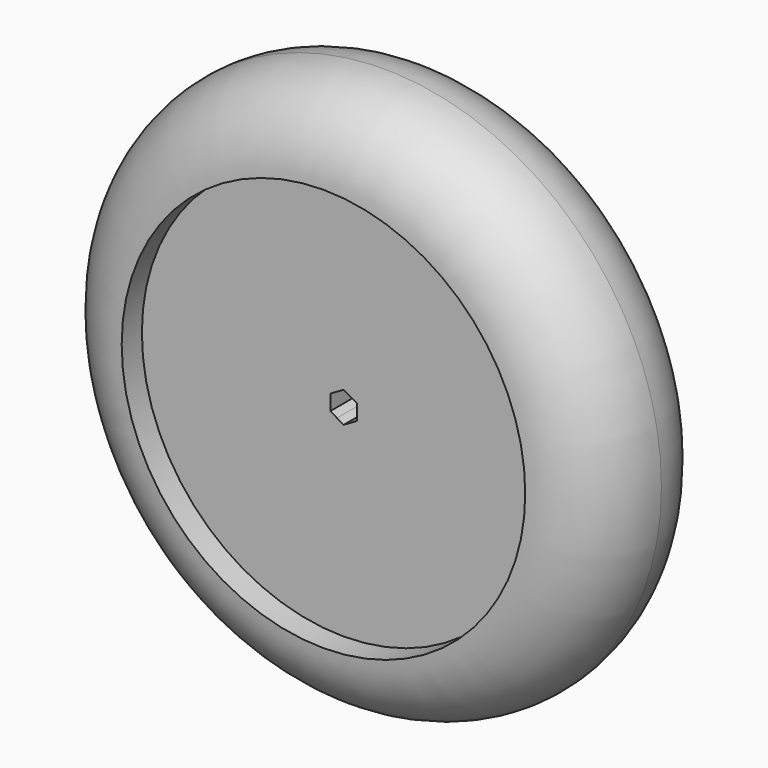
from build123d import *

# Parameters (mm, degrees)
F0_R     = 27.5
F1_DEPTH = 7.5
F2_R     = 7.49999
F3_DEPTH = 2.5
F4_DEPTH = 5


# Not quite as in the source:
# - a fillet or chamfer is up to 0.001 mm smaller than in the source, because OpenCascade refuses the exact size


with BuildPart() as f1:
    # F0 (on Front) → F1 (new body, symmetric)
    with BuildSketch(Plane.XZ):
        Circle(F0_R)
        Polygon((1.325, 0.7649891067), (1.325, 0), (1.325, -0.7649891067), (0.6624999921, -1.1474836645), (0, -1.5299782134), (-0.6624999921, -1.1474836645), (-1.325, -0.7649891067), (-1.325, 0), (-1.325, 0.7649891067), (-0.6624999921, 1.1474836645), (0, 1.5299782134), (0.6624999921, 1.1474836645), align=None, mode=Mode.SUBTRACT)
    extrude(amount=F1_DEPTH, both=True)

    # F2 (radius 7.5 in the source; OpenCascade refuses exactly that, so slightly less here)
    f2_edges = [f1.edges().sort_by_distance(p)[0] for p in [
        (-27.5, -7.5, 0),
        (-27.5, 7.5, 0),
    ]]
    fillet(f2_edges, radius=F2_R)

    # F3 (cut, symmetric): a face of the model
    f3_faces = [f1.faces().sort_by_distance(p)[0] for p in [
        (-19.4343242922, -7.5, 0),
    ]]
    extrude(f3_faces, amount=F3_DEPTH, both=True, mode=Mode.SUBTRACT)

    # F4 (cut): a face of the model
    f4_faces = [f1.faces().sort_by_distance(p)[0] for p in [
        (-19.4343242922, 7.5, 0),
    ]]
    extrude(f4_faces, amount=-F4_DEPTH, mode=Mode.SUBTRACT)


solid = f1.part
